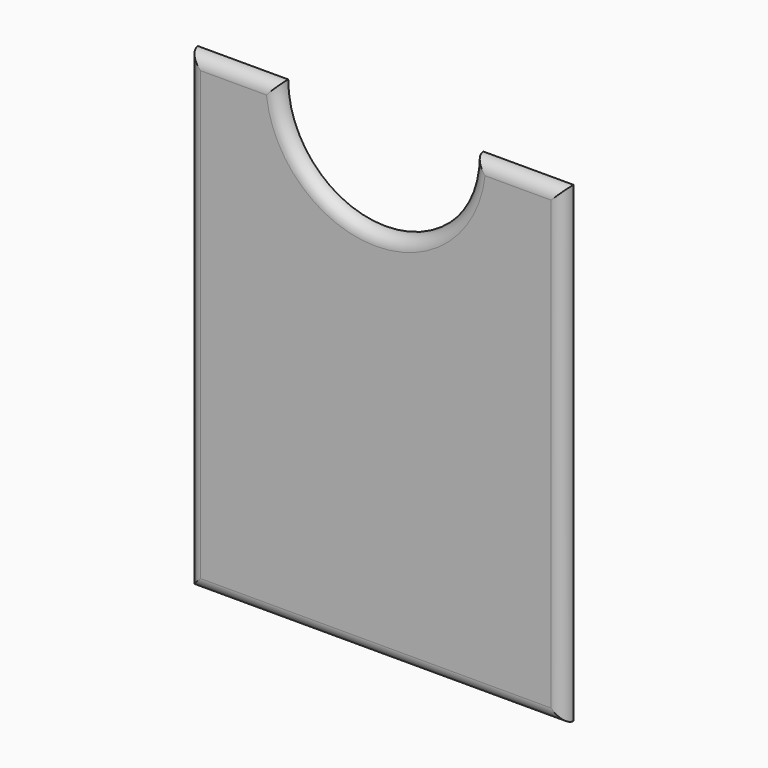
from build123d import *

# Parameters (mm, degrees)
F1_DEPTH = 5.08
F2_R     = 5.07999


# Not quite as in the source:
# - a fillet or chamfer is up to 0.001 mm smaller than in the source, because OpenCascade refuses the exact size


with BuildPart() as f1:
    # F0 (on Front) → F1 (new body)
    with BuildSketch(Plane.XZ):
        with BuildLine():
            Line((76.3972327113, 76.3972327113), (39.6787461365, 76.3972327113))
            ThreePointArc((39.6787461365, 76.3972327113), (3.7253e-06, 36.7184903001), (-39.678738686, 76.3972327113))
            Line((-39.678738686, 76.3972327113), (-76.3972252607, 76.3972327113))
            Line((-76.3972252607, 76.3972327113), (-76.3972252607, -115.6601980329))
            Line((-76.3972252607, -115.6601980329), (76.3972327113, -115.6601980329))
            Line((76.3972327113, -115.6601980329), (76.3972327113, 76.3972327113))
        make_face()
    extrude(amount=F1_DEPTH)

    # F2 (radius 5.08 in the source; OpenCascade refuses exactly that, so slightly less here)
    f2_edges = [f1.edges().sort_by_distance(p)[0] for p in [
        (-58.037982, -5.08, 76.397233),
        (-76.397225, -5.08, -19.631483),
        (4e-06, -5.08, 36.71849),
        (58.037989, -5.08, 76.397233),
        (76.397233, -5.08, -19.631483),
        (4e-06, -5.08, -115.660198),
    ]]
    fillet(f2_edges, radius=F2_R)


solid = f1.part
